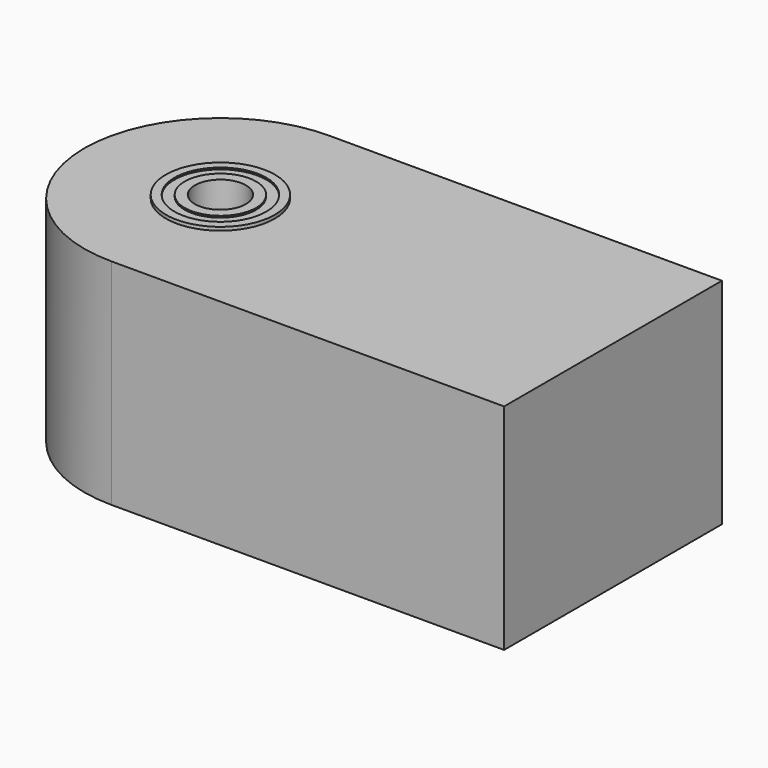
from build123d import *

# Parameters (mm, degrees)
F0_R     = 16
F0_R_2   = 13.5
F1_DEPTH = 9
F0_R_3   = 10.5
F0_R_4   = 7.5
F2_DEPTH = 8.5
F3_DEPTH = 0.5
F4_R     = 16
F5_DEPTH = 8
F4_R_2   = 10.5
F6_DEPTH = 55


with BuildPart() as f1:
    # F0 (on Top) → F1 (new body)
    with BuildSketch(Plane.XY):
        Circle(F0_R)
        Circle(F0_R_2, mode=Mode.SUBTRACT)
    extrude(amount=F1_DEPTH)


with BuildPart() as f1b:
    # F0 (on Top) → F1, piece 2 (new body)
    with BuildSketch(Plane.XY):
        Circle(F0_R_3)
        Circle(F0_R_4, mode=Mode.SUBTRACT)
    extrude(amount=F1_DEPTH)


with BuildPart() as f2:
    # F0 (on Top) → F2 (new body)
    with BuildSketch(Plane.XY):
        Circle(F0_R_2)
        Circle(F0_R_3, mode=Mode.SUBTRACT)
    extrude(amount=F2_DEPTH)

    # F3 (cut): a face of the model
    f3_faces = [f2.faces().sort_by_distance(p)[0] for p in [
        (-13.1181623382, 0, 0),
    ]]
    extrude(f3_faces, amount=-F3_DEPTH, mode=Mode.SUBTRACT)


with BuildPart() as f5:
    # F4 (on Top) → F5 (new body)
    with BuildSketch(Plane.XY):
        with BuildLine():
            Line((115.3682768345, 40), (0, 40))
            ThreePointArc((0, 40), (-40, 0), (0, -40))
            Line((0, -40), (115.3682768345, -40))
            Line((115.3682768345, -40), (115.3682768345, 40))
        make_face()
        Circle(F4_R, mode=Mode.SUBTRACT)
    extrude(amount=F5_DEPTH)

    # F4 (on Top) → F6 (join)
    with BuildSketch(Plane.XY):
        with BuildLine():
            Line((115.3682768345, 40), (0, 40))
            ThreePointArc((0, 40), (-40, 0), (0, -40))
            Line((0, -40), (115.3682768345, -40))
            Line((115.3682768345, -40), (115.3682768345, 40))
        make_face()
        Circle(F4_R, mode=Mode.SUBTRACT)
        Circle(F4_R)
        Circle(F4_R_2, mode=Mode.SUBTRACT)
    extrude(amount=-F6_DEPTH)


solid = Compound([f1.part, f1b.part, f2.part, f5.part])
